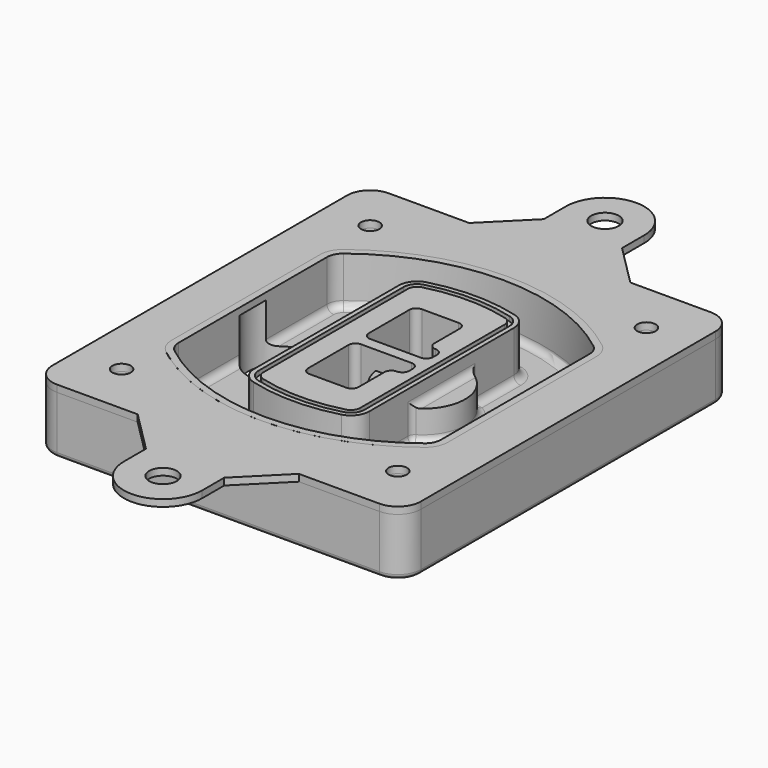
from build123d import *

# Parameters (mm, degrees)
F0_R      = 4
F1_DEPTH  = 25
F2_DEPTH  = 3
F3_DEPTH  = 18
F5_DEPTH  = 21
F6_DEPTH  = 2
F8_DEPTH  = 20
F9_DEPTH  = 16
F10_DEPTH = 25
F7_R      = 6
F7_R_2    = 4
F11_DEPTH = 6
F13_DEPTH = 9
F14_R     = 3
F15_R     = 2
F16_R     = 4
F16_R_2   = 6
F17_DEPTH = 3


with BuildPart() as f1:
    # F0 (on Top) → F1 (new body)
    with BuildSketch(Plane.XY):
        with BuildLine():
            ThreePointArc((-80, -80), (-77.0710678119, -87.0710678119), (-70, -90))
            Line((-70, -90), (70, -90))
            ThreePointArc((70, -90), (77.0710678119, -87.0710678119), (80, -80))
            Line((80, -80), (80, 80))
            ThreePointArc((80, 80), (77.0710678119, 87.0710678119), (70, 90))
            Line((70, 90), (-70, 90))
            ThreePointArc((-70, 90), (-77.0710678119, 87.0710678119), (-80, 80))
            Line((-80, 80), (-80, -80))
        make_face()
        with Locations((-60, -67.5)):
            Circle(F0_R, mode=Mode.SUBTRACT)
        with Locations((60, -67.5)):
            Circle(F0_R, mode=Mode.SUBTRACT)
        with Locations((-60, 67.5)):
            Circle(F0_R, mode=Mode.SUBTRACT)
        with BuildLine():
            ThreePointArc((-64, 40.2934422872), (-62.5820384798, 46.4328484224), (-58.6153846154, 51.3286200352))
            ThreePointArc((-58.6153846154, 51.3286200352), (0, 71.5), (58.6153846154, 51.3286200352))
            ThreePointArc((58.6153846154, 51.3286200352), (62.5820384798, 46.4328484224), (64, 40.2934422872))
            Line((64, 40.2934422872), (64, -40.2934422872))
            ThreePointArc((64, -40.2934422872), (62.5820384798, -46.4328484224), (58.6153846154, -51.3286200352))
            ThreePointArc((58.6153846154, -51.3286200352), (0, -71.5), (-58.6153846154, -51.3286200352))
            ThreePointArc((-58.6153846154, -51.3286200352), (-62.5820384798, -46.4328484224), (-64, -40.2934422872))
            Line((-64, -40.2934422872), (-64, 40.2934422872))
        make_face(mode=Mode.SUBTRACT)
        with Locations((60, 67.5)):
            Circle(F0_R, mode=Mode.SUBTRACT)
        with BuildLine():
            ThreePointArc((58.6153846154, 51.3286200352), (0, 71.5), (-58.6153846154, 51.3286200352))
            ThreePointArc((-58.6153846154, 51.3286200352), (-62.5820384798, 46.4328484224), (-64, 40.2934422872))
            Line((-64, 40.2934422872), (-64, -40.2934422872))
            ThreePointArc((-64, -40.2934422872), (-62.5820384798, -46.4328484224), (-58.6153846154, -51.3286200352))
            ThreePointArc((-58.6153846154, -51.3286200352), (0, -71.5), (58.6153846154, -51.3286200352))
            ThreePointArc((58.6153846154, -51.3286200352), (62.5820384798, -46.4328484224), (64, -40.2934422872))
            Line((64, -40.2934422872), (64, 40.2934422872))
            ThreePointArc((64, 40.2934422872), (62.5820384798, 46.4328484224), (58.6153846154, 51.3286200352))
        make_face()
        with BuildLine():
            Line((-60, -40.2934422872), (-60, 40.2934422872))
            ThreePointArc((-60, 40.2934422872), (-58.9871703427, 44.6787323838), (-56.1538461538, 48.1757121072))
            ThreePointArc((-56.1538461538, 48.1757121072), (0, 67.5), (56.1538461538, 48.1757121072))
            ThreePointArc((56.1538461538, 48.1757121072), (58.9871703427, 44.6787323838), (60, 40.2934422872))
            Line((60, 40.2934422872), (60, -40.2934422872))
            ThreePointArc((60, -40.2934422872), (58.9871703427, -44.6787323838), (56.1538461538, -48.1757121072))
            ThreePointArc((56.1538461538, -48.1757121072), (0, -67.5), (-56.1538461538, -48.1757121072))
            ThreePointArc((-56.1538461538, -48.1757121072), (-58.9871703427, -44.6787323838), (-60, -40.2934422872))
        make_face(mode=Mode.SUBTRACT)
        with BuildLine():
            ThreePointArc((-56.1538461538, 48.1757121072), (-58.9871703427, 44.6787323838), (-60, 40.2934422872))
            Line((-60, 40.2934422872), (-60, -40.2934422872))
            ThreePointArc((-60, -40.2934422872), (-58.9871703427, -44.6787323838), (-56.1538461538, -48.1757121072))
            ThreePointArc((-56.1538461538, -48.1757121072), (0, -67.5), (56.1538461538, -48.1757121072))
            ThreePointArc((56.1538461538, -48.1757121072), (58.9871703427, -44.6787323838), (60, -40.2934422872))
            Line((60, -40.2934422872), (60, 40.2934422872))
            ThreePointArc((60, 40.2934422872), (58.9871703427, 44.6787323838), (56.1538461538, 48.1757121072))
            ThreePointArc((56.1538461538, 48.1757121072), (0, 67.5), (-56.1538461538, 48.1757121072))
        make_face()
        with BuildLine():
            ThreePointArc((54.3076923077, 45.8110311612), (56.2910192399, 43.3631453548), (57, 40.2934422872))
            Line((57, 40.2934422872), (57, -40.2934422872))
            ThreePointArc((57, -40.2934422872), (56.2910192399, -43.3631453548), (54.3076923077, -45.8110311612))
            ThreePointArc((54.3076923077, -45.8110311612), (0, -64.5), (-54.3076923077, -45.8110311612))
            ThreePointArc((-54.3076923077, -45.8110311612), (-56.2910192399, -43.3631453548), (-57, -40.2934422872))
            Line((-57, -40.2934422872), (-57, 40.2934422872))
            ThreePointArc((-57, 40.2934422872), (-56.2910192399, 43.3631453548), (-54.3076923077, 45.8110311612))
            ThreePointArc((-54.3076923077, 45.8110311612), (0, 64.5), (54.3076923077, 45.8110311612))
        make_face(mode=Mode.SUBTRACT)
        with BuildLine():
            Line((57, -40.2934422872), (57, 40.2934422872))
            ThreePointArc((57, 40.2934422872), (56.2910192399, 43.3631453548), (54.3076923077, 45.8110311612))
            ThreePointArc((54.3076923077, 45.8110311612), (0, 64.5), (-54.3076923077, 45.8110311612))
            ThreePointArc((-54.3076923077, 45.8110311612), (-56.2910192399, 43.3631453548), (-57, 40.2934422872))
            Line((-57, 40.2934422872), (-57, -40.2934422872))
            ThreePointArc((-57, -40.2934422872), (-56.2910192399, -43.3631453548), (-54.3076923077, -45.8110311612))
            ThreePointArc((-54.3076923077, -45.8110311612), (0, -64.5), (54.3076923077, -45.8110311612))
            ThreePointArc((54.3076923077, -45.8110311612), (56.2910192399, -43.3631453548), (57, -40.2934422872))
        make_face()
    extrude(amount=-F1_DEPTH)

    # F0 (on Top) → F2 (join)
    with BuildSketch(Plane.XY):
        with BuildLine():
            ThreePointArc((-56.1538461538, 48.1757121072), (-58.9871703427, 44.6787323838), (-60, 40.2934422872))
            Line((-60, 40.2934422872), (-60, -40.2934422872))
            ThreePointArc((-60, -40.2934422872), (-58.9871703427, -44.6787323838), (-56.1538461538, -48.1757121072))
            ThreePointArc((-56.1538461538, -48.1757121072), (0, -67.5), (56.1538461538, -48.1757121072))
            ThreePointArc((56.1538461538, -48.1757121072), (58.9871703427, -44.6787323838), (60, -40.2934422872))
            Line((60, -40.2934422872), (60, 40.2934422872))
            ThreePointArc((60, 40.2934422872), (58.9871703427, 44.6787323838), (56.1538461538, 48.1757121072))
            ThreePointArc((56.1538461538, 48.1757121072), (0, 67.5), (-56.1538461538, 48.1757121072))
        make_face()
        with BuildLine():
            ThreePointArc((54.3076923077, 45.8110311612), (56.2910192399, 43.3631453548), (57, 40.2934422872))
            Line((57, 40.2934422872), (57, -40.2934422872))
            ThreePointArc((57, -40.2934422872), (56.2910192399, -43.3631453548), (54.3076923077, -45.8110311612))
            ThreePointArc((54.3076923077, -45.8110311612), (0, -64.5), (-54.3076923077, -45.8110311612))
            ThreePointArc((-54.3076923077, -45.8110311612), (-56.2910192399, -43.3631453548), (-57, -40.2934422872))
            Line((-57, -40.2934422872), (-57, 40.2934422872))
            ThreePointArc((-57, 40.2934422872), (-56.2910192399, 43.3631453548), (-54.3076923077, 45.8110311612))
            ThreePointArc((-54.3076923077, 45.8110311612), (0, 64.5), (54.3076923077, 45.8110311612))
        make_face(mode=Mode.SUBTRACT)
    extrude(amount=F2_DEPTH)

    # F0 (on Top) → F3 (cut)
    with BuildSketch(Plane.XY):
        with BuildLine():
            Line((57, -40.2934422872), (57, 40.2934422872))
            ThreePointArc((57, 40.2934422872), (56.2910192399, 43.3631453548), (54.3076923077, 45.8110311612))
            ThreePointArc((54.3076923077, 45.8110311612), (0, 64.5), (-54.3076923077, 45.8110311612))
            ThreePointArc((-54.3076923077, 45.8110311612), (-56.2910192399, 43.3631453548), (-57, 40.2934422872))
            Line((-57, 40.2934422872), (-57, -40.2934422872))
            ThreePointArc((-57, -40.2934422872), (-56.2910192399, -43.3631453548), (-54.3076923077, -45.8110311612))
            ThreePointArc((-54.3076923077, -45.8110311612), (0, -64.5), (54.3076923077, -45.8110311612))
            ThreePointArc((54.3076923077, -45.8110311612), (56.2910192399, -43.3631453548), (57, -40.2934422872))
        make_face()
    extrude(amount=-F3_DEPTH, mode=Mode.SUBTRACT)

    # F4 (on face) → F5 (join, through all)
    with BuildSketch(Plane.XY.offset(3)):
        with BuildLine():
            ThreePointArc((-25, -39.2465276821), (-23.3511545998, -44.1109737193), (-19.0842911877, -46.9702398883))
            ThreePointArc((-19.0842911877, -46.9702398883), (0, -49.5), (19.0842911877, -46.9702398883))
            ThreePointArc((19.0842911877, -46.9702398883), (23.3511545998, -44.1109737193), (25, -39.2465276821))
            Line((25, -39.2465276821), (25, 39.2465276821))
            ThreePointArc((25, 39.2465276821), (23.3511545998, 44.1109737193), (19.0842911877, 46.9702398883))
            ThreePointArc((19.0842911877, 46.9702398883), (0, 49.5), (-19.0842911877, 46.9702398883))
            ThreePointArc((-19.0842911877, 46.9702398883), (-23.3511545998, 44.1109737193), (-25, 39.2465276821))
            Line((-25, 39.2465276821), (-25, -39.2465276821))
        make_face()
        with BuildLine():
            ThreePointArc((18.5632183908, 45.0393118368), (21.7633659499, 42.89486221), (23, 39.2465276821))
            Line((23, 39.2465276821), (23, -39.2465276821))
            ThreePointArc((23, -39.2465276821), (21.7633659499, -42.89486221), (18.5632183908, -45.0393118368))
            ThreePointArc((18.5632183908, -45.0393118368), (0, -47.5), (-18.5632183908, -45.0393118368))
            ThreePointArc((-18.5632183908, -45.0393118368), (-21.7633659499, -42.89486221), (-23, -39.2465276821))
            Line((-23, -39.2465276821), (-23, 39.2465276821))
            ThreePointArc((-23, 39.2465276821), (-21.7633659499, 42.89486221), (-18.5632183908, 45.0393118368))
            ThreePointArc((-18.5632183908, 45.0393118368), (0, 47.5), (18.5632183908, 45.0393118368))
        make_face(mode=Mode.SUBTRACT)
        with BuildLine():
            Line((23, -39.2465276821), (23, 39.2465276821))
            ThreePointArc((23, 39.2465276821), (21.7633659499, 42.89486221), (18.5632183908, 45.0393118368))
            ThreePointArc((18.5632183908, 45.0393118368), (0, 47.5), (-18.5632183908, 45.0393118368))
            ThreePointArc((-18.5632183908, 45.0393118368), (-21.7633659499, 42.89486221), (-23, 39.2465276821))
            Line((-23, 39.2465276821), (-23, -39.2465276821))
            ThreePointArc((-23, -39.2465276821), (-21.7633659499, -42.89486221), (-18.5632183908, -45.0393118368))
            ThreePointArc((-18.5632183908, -45.0393118368), (0, -47.5), (18.5632183908, -45.0393118368))
            ThreePointArc((18.5632183908, -45.0393118368), (21.7633659499, -42.89486221), (23, -39.2465276821))
        make_face()
        with BuildLine():
            ThreePointArc((18.0421455939, 43.1083837852), (20.1755772999, 41.6787507007), (21, 39.2465276821))
            Line((21, 39.2465276821), (21, -39.2465276821))
            ThreePointArc((21, -39.2465276821), (20.1755772999, -41.6787507007), (18.0421455939, -43.1083837852))
            ThreePointArc((18.0421455939, -43.1083837852), (0, -45.5), (-18.0421455939, -43.1083837852))
            ThreePointArc((-18.0421455939, -43.1083837852), (-20.1755772999, -41.6787507007), (-21, -39.2465276821))
            Line((-21, -39.2465276821), (-21, 39.2465276821))
            ThreePointArc((-21, 39.2465276821), (-20.1755772999, 41.6787507007), (-18.0421455939, 43.1083837852))
            ThreePointArc((-18.0421455939, 43.1083837852), (0, 45.5), (18.0421455939, 43.1083837852))
        make_face(mode=Mode.SUBTRACT)
        with BuildLine():
            Line((21, -39.2465276821), (21, 39.2465276821))
            ThreePointArc((21, 39.2465276821), (20.1755772999, 41.6787507007), (18.0421455939, 43.1083837852))
            ThreePointArc((18.0421455939, 43.1083837852), (0, 45.5), (-18.0421455939, 43.1083837852))
            ThreePointArc((-18.0421455939, 43.1083837852), (-20.1755772999, 41.6787507007), (-21, 39.2465276821))
            Line((-21, 39.2465276821), (-21, -39.2465276821))
            ThreePointArc((-21, -39.2465276821), (-20.1755772999, -41.6787507007), (-18.0421455939, -43.1083837852))
            ThreePointArc((-18.0421455939, -43.1083837852), (0, -45.5), (18.0421455939, -43.1083837852))
            ThreePointArc((18.0421455939, -43.1083837852), (20.1755772999, -41.6787507007), (21, -39.2465276821))
        make_face()
        with BuildLine():
            Line((-8, -2.5), (14, -2.5))
            ThreePointArc((14, -2.5), (16.1213203436, -3.3786796564), (17, -5.5))
            Line((17, -5.5), (17, -7.5))
            ThreePointArc((17, -7.5), (16.1213203436, -9.6213203436), (14, -10.5))
            ThreePointArc((14, -10.5), (11.8786796564, -11.3786796564), (11, -13.5))
            Line((11, -13.5), (11, -27.5))
            ThreePointArc((11, -27.5), (10.1213203436, -29.6213203436), (8, -30.5))
            Line((8, -30.5), (-8, -30.5))
            ThreePointArc((-8, -30.5), (-10.1213203436, -29.6213203436), (-11, -27.5))
            Line((-11, -27.5), (-11, -5.5))
            ThreePointArc((-11, -5.5), (-10.1213203436, -3.3786796564), (-8, -2.5))
        make_face(mode=Mode.SUBTRACT)
        with BuildLine():
            ThreePointArc((-8, 2.5), (-10.1213203436, 3.3786796564), (-11, 5.5))
            Line((-11, 5.5), (-11, 27.5))
            ThreePointArc((-11, 27.5), (-10.1213203436, 29.6213203436), (-8, 30.5))
            Line((-8, 30.5), (8, 30.5))
            ThreePointArc((8, 30.5), (10.1213203436, 29.6213203436), (11, 27.5))
            Line((11, 27.5), (11, 13.5))
            ThreePointArc((11, 13.5), (11.8786796564, 11.3786796564), (14, 10.5))
            ThreePointArc((14, 10.5), (16.1213203436, 9.6213203436), (17, 7.5))
            Line((17, 7.5), (17, 5.5))
            ThreePointArc((17, 5.5), (16.1213203436, 3.3786796564), (14, 2.5))
            Line((14, 2.5), (-8, 2.5))
        make_face(mode=Mode.SUBTRACT)
    extrude(amount=-F5_DEPTH)

    # F4 (on face) → F6 (cut)
    with BuildSketch(Plane.XY.offset(3)):
        with BuildLine():
            Line((23, -39.2465276821), (23, 39.2465276821))
            ThreePointArc((23, 39.2465276821), (21.7633659499, 42.89486221), (18.5632183908, 45.0393118368))
            ThreePointArc((18.5632183908, 45.0393118368), (0, 47.5), (-18.5632183908, 45.0393118368))
            ThreePointArc((-18.5632183908, 45.0393118368), (-21.7633659499, 42.89486221), (-23, 39.2465276821))
            Line((-23, 39.2465276821), (-23, -39.2465276821))
            ThreePointArc((-23, -39.2465276821), (-21.7633659499, -42.89486221), (-18.5632183908, -45.0393118368))
            ThreePointArc((-18.5632183908, -45.0393118368), (0, -47.5), (18.5632183908, -45.0393118368))
            ThreePointArc((18.5632183908, -45.0393118368), (21.7633659499, -42.89486221), (23, -39.2465276821))
        make_face()
        with BuildLine():
            ThreePointArc((18.0421455939, 43.1083837852), (20.1755772999, 41.6787507007), (21, 39.2465276821))
            Line((21, 39.2465276821), (21, -39.2465276821))
            ThreePointArc((21, -39.2465276821), (20.1755772999, -41.6787507007), (18.0421455939, -43.1083837852))
            ThreePointArc((18.0421455939, -43.1083837852), (0, -45.5), (-18.0421455939, -43.1083837852))
            ThreePointArc((-18.0421455939, -43.1083837852), (-20.1755772999, -41.6787507007), (-21, -39.2465276821))
            Line((-21, -39.2465276821), (-21, 39.2465276821))
            ThreePointArc((-21, 39.2465276821), (-20.1755772999, 41.6787507007), (-18.0421455939, 43.1083837852))
            ThreePointArc((-18.0421455939, 43.1083837852), (0, 45.5), (18.0421455939, 43.1083837852))
        make_face(mode=Mode.SUBTRACT)
    extrude(amount=-F6_DEPTH, mode=Mode.SUBTRACT)

    # F7 (on face) → F8 (join)
    with BuildSketch(Plane(origin=(0, 0, -25), x_dir=(1, 0, 0), z_dir=(0, 0, -1))):
        with BuildLine():
            ThreePointArc((3.28842436, 0), (16.7567035675, 13.4682792075), (30.224982775, 0))
            Line((30.224982775, 0), (35.224982775, 0))
            ThreePointArc((35.224982775, 0), (16.7567035675, 18.4682792075), (-1.71157564, 0))
            Line((-1.71157564, 0), (3.28842436, 0))
        make_face()
        with BuildLine():
            Line((3.28842436, 0), (30.224982775, 0))
            ThreePointArc((30.224982775, 0), (16.7567035675, 13.4682792075), (3.28842436, 0))
        make_face()
        with BuildLine():
            ThreePointArc((3.28842436, 0), (16.7567035675, -13.4682792075), (30.224982775, 0))
            Line((30.224982775, 0), (3.28842436, 0))
        make_face()
        with BuildLine():
            Line((35.224982775, 0), (30.224982775, 0))
            ThreePointArc((30.224982775, 0), (16.7567035675, -13.4682792075), (3.28842436, 0))
            Line((3.28842436, 0), (-1.71157564, 0))
            ThreePointArc((-1.71157564, 0), (16.7567035675, -18.4682792075), (35.224982775, 0))
        make_face()
    extrude(amount=-F8_DEPTH)

    # F7 (on face) → F9 (cut)
    with BuildSketch(Plane(origin=(0, 0, -25), x_dir=(1, 0, 0), z_dir=(0, 0, -1))):
        with BuildLine():
            Line((3.28842436, 0), (30.224982775, 0))
            ThreePointArc((30.224982775, 0), (16.7567035675, 13.4682792075), (3.28842436, 0))
        make_face()
        with BuildLine():
            ThreePointArc((3.28842436, 0), (16.7567035675, -13.4682792075), (30.224982775, 0))
            Line((30.224982775, 0), (3.28842436, 0))
        make_face()
    extrude(amount=-F9_DEPTH, mode=Mode.SUBTRACT)

    # F7 (on face) → F10 (cut)
    with BuildSketch(Plane(origin=(0, 0, -25), x_dir=(1, 0, 0), z_dir=(0, 0, -1))):
        with BuildLine():
            Line((-59.0318229325, 0), (-32.0952645175, 0))
            ThreePointArc((-32.0952645175, 0), (-45.563543725, 13.4682792075), (-59.0318229325, 0))
        make_face()
        with BuildLine():
            ThreePointArc((-59.0318229325, 0), (-45.563543725, -13.4682792075), (-32.0952645175, 0))
            Line((-32.0952645175, 0), (-59.0318229325, 0))
        make_face()
    extrude(amount=-F10_DEPTH, mode=Mode.SUBTRACT)

    # F7 (on face) → F11 (cut)
    with BuildSketch(Plane(origin=(0, 0, -25), x_dir=(1, 0, 0), z_dir=(0, 0, -1))):
        with Locations((60, -67.5)):
            Circle(F7_R)
        with Locations((60, -67.5)):
            Circle(F7_R_2, mode=Mode.SUBTRACT)
        with Locations((-60, -67.5)):
            Circle(F7_R)
        with Locations((-60, -67.5)):
            Circle(F7_R_2, mode=Mode.SUBTRACT)
        with Locations((-60, 67.5)):
            Circle(F7_R)
        with Locations((-60, 67.5)):
            Circle(F7_R_2, mode=Mode.SUBTRACT)
        with Locations((60, 67.5)):
            Circle(F7_R)
        with Locations((60, 67.5)):
            Circle(F7_R_2, mode=Mode.SUBTRACT)
    extrude(amount=-F11_DEPTH, mode=Mode.SUBTRACT)

    # F12 (on face) → F13 (cut, through all)
    with BuildSketch(Plane(origin=(0, 0, -9), x_dir=(1, 0, 0), z_dir=(0, 0, -1))):
        with BuildLine():
            Line((11, 13.5), (11, 17.5481537753))
            ThreePointArc((11, 17.5481537753), (2.5696536419, 11.8239143813), (-1.5415842455, 2.5))
            Line((-1.5415842455, 2.5), (3.5224848595, 2.5))
            ThreePointArc((3.5224848595, 2.5), (6.1857188154, 8.3455872281), (11.2536447004, 12.2927168648))
            ThreePointArc((11.2536447004, 12.2927168648), (11.0640958889, 12.8831798879), (11, 13.5))
        make_face()
        with BuildLine():
            ThreePointArc((11.2536447004, -12.2927168648), (6.1857188154, -8.3455872281), (3.5224848595, -2.5))
            Line((3.5224848595, -2.5), (-1.5415842455, -2.5))
            ThreePointArc((-1.5415842455, -2.5), (2.5696536419, -11.8239143813), (11, -17.5481537753))
            Line((11, -17.5481537753), (11, -13.5))
            ThreePointArc((11, -13.5), (11.0640958889, -12.8831798879), (11.2536447004, -12.2927168648))
        make_face()
        with BuildLine():
            ThreePointArc((11.2536447004, 12.2927168648), (6.1857188154, 8.3455872281), (3.5224848595, 2.5))
            Line((3.5224848595, 2.5), (14, 2.5))
            ThreePointArc((14, 2.5), (16.1213203436, 3.3786796564), (17, 5.5))
            Line((17, 5.5), (17, 7.5))
            ThreePointArc((17, 7.5), (16.1213203436, 9.6213203436), (14, 10.5))
            ThreePointArc((14, 10.5), (12.3601599782, 10.9878446101), (11.2536447004, 12.2927168648))
        make_face()
        with BuildLine():
            Line((14, -2.5), (3.5224848595, -2.5))
            ThreePointArc((3.5224848595, -2.5), (6.1857188154, -8.3455872281), (11.2536447004, -12.2927168648))
            ThreePointArc((11.2536447004, -12.2927168648), (12.3601599782, -10.9878446101), (14, -10.5))
            ThreePointArc((14, -10.5), (16.1213203436, -9.6213203436), (17, -7.5))
            Line((17, -7.5), (17, -5.5))
            ThreePointArc((17, -5.5), (16.1213203436, -3.3786796564), (14, -2.5))
        make_face()
    extrude(amount=F13_DEPTH, mode=Mode.SUBTRACT)

    # F14
    f14_edges = [f1.edges().sort_by_distance(p)[0] for p in [
        (-57, -23.703476, -18),
        (-57, 23.703476, -18),
        (25, 0, -5),
        (25, 16.526506, -11.5),
        (25, -16.526506, -11.5),
        (25, -27.886517, -18),
        (35.224983, 0, -18),
    ]]
    fillet(f14_edges, radius=F14_R)

    # F15
    f15_edges = [f1.edges().sort_by_distance(p)[0] for p in [
        (0, -90, -25),
    ]]
    fillet(f15_edges, radius=F15_R)


with BuildPart() as f17:
    # F16 (on face) → F17 (new body, through all)
    with BuildSketch(Plane.XY):
        with BuildLine():
            Line((-35, 90), (-70, 90))
            ThreePointArc((-70, 90), (-77.0710678119, 87.0710678119), (-80, 80))
            Line((-80, 80), (-80, -60.79364568))
            Line((-80, -60.79364568), (-80, -80))
            ThreePointArc((-80, -80), (-77.0710678119, -87.0710678119), (-70, -90))
            Line((-70, -90), (-35, -90))
            Line((-35, -90), (35, -90))
            Line((35, -90), (60.4784972966, -90))
            Line((60.4784972966, -90), (70, -90))
            ThreePointArc((70, -90), (77.0710678119, -87.0710678119), (80, -80))
            Line((80, -80), (80, -62.2497312725))
            Line((80, -62.2497312725), (80, 62.2457452118))
            Line((80, 62.2457452118), (80, 80))
            ThreePointArc((80, 80), (77.0710678119, 87.0710678119), (70, 90))
            Line((70, 90), (36.9651950896, 90))
            Line((36.9651950896, 90), (35, 90))
            Line((35, 90), (0, 90))
            Line((0, 90), (-35, 90))
        make_face()
        with Locations((-60, -67.5)):
            Circle(F16_R, mode=Mode.SUBTRACT)
        with Locations((60, -67.5)):
            Circle(F16_R, mode=Mode.SUBTRACT)
        with Locations((-60, 67.5)):
            Circle(F16_R, mode=Mode.SUBTRACT)
        with BuildLine():
            ThreePointArc((-56.1538461538, 48.1757121072), (0, 67.5), (56.1538461538, 48.1757121072))
            ThreePointArc((56.1538461538, 48.1757121072), (58.9871703427, 44.6787323838), (60, 40.2934422872))
            Line((60, 40.2934422872), (60, -40.2934422872))
            ThreePointArc((60, -40.2934422872), (58.9871703427, -44.6787323838), (56.1538461538, -48.1757121072))
            ThreePointArc((56.1538461538, -48.1757121072), (2.5461394088, -67.4644707495), (-52.0540978471, -51.196203355))
            ThreePointArc((-52.0540978471, -51.196203355), (-54.1250462177, -49.7145620141), (-56.1538461538, -48.1757121072))
            ThreePointArc((-56.1538461538, -48.1757121072), (-58.9871703427, -44.6787323838), (-60, -40.2934422872))
            Line((-60, -40.2934422872), (-60, 40.2934422872))
            ThreePointArc((-60, 40.2934422872), (-58.9871703427, 44.6787323838), (-56.1538461538, 48.1757121072))
        make_face(mode=Mode.SUBTRACT)
        with Locations((60, 67.5)):
            Circle(F16_R, mode=Mode.SUBTRACT)
        with BuildLine():
            Line((-17, 108), (-35, 90))
            Line((-35, 90), (0, 90))
            Line((0, 90), (35, 90))
            Line((35, 90), (17, 108))
            Line((17, 108), (17, 120))
            ThreePointArc((17, 120), (0, 137), (-17, 120))
            Line((-17, 120), (-17, 108))
        make_face()
        with Locations((0, 120)):
            Circle(F16_R_2, mode=Mode.SUBTRACT)
        with BuildLine():
            Line((35, -90), (-35, -90))
            Line((-35, -90), (-17, -108))
            Line((-17, -108), (-17, -120))
            ThreePointArc((-17, -120), (0, -137), (17, -120))
            Line((17, -120), (17, -108))
            Line((17, -108), (35, -90))
        make_face()
        with Locations((0, -120)):
            Circle(F16_R_2, mode=Mode.SUBTRACT)
    extrude(amount=F17_DEPTH)


solid = Compound([f1.part, f17.part])
